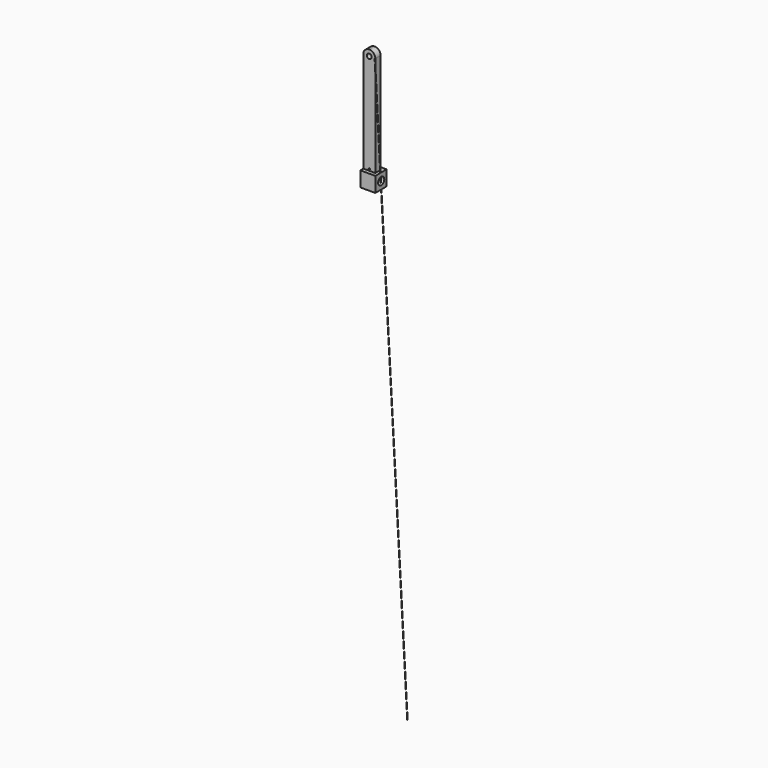
from build123d import *
from build123d import SkipClean  # not in build123d's __all__

# Parameters (mm, degrees)
F1_DEPTH      = 22
F2_R          = 8.15
F3_DEPTH      = 22.001
F3_TAPER      = 5.72
F4_W          = 40
F4_H          = 50
F5_DEPTH      = 12.5
F5_DEPTH_BACK = 34.5
F6_R          = 12.7
F7_DEPTH      = 40.001
F8_R          = 12.7
F9_DEPTH      = 10
F10_R         = 2.5
F11_DEPTH     = 25
F14_R         = 0.5
F15_DEPTH     = 2000


# Not quite as in the source:
# - after a boolean that leaves OpenCascade's solid faulty, fix() repairs it


with BuildPart() as f1:
    # F0 (on Front) → F1 (new body)
    with BuildSketch(Plane.XZ):
        with BuildLine():
            Line((0, 385), (0, 0))
            Line((0, 0), (40, 0))
            Line((40, 0), (40, 385))
            ThreePointArc((40, 385), (34.1421356237, 399.1421356237), (20, 405))
            ThreePointArc((20, 405), (5.8578643763, 399.1421356237), (0, 385))
        make_face()
    extrude(amount=F1_DEPTH)

    # F2 (on face) → F3 (cut, through all)
    with BuildSketch(Plane.XZ.offset(22)):
        with Locations((20, 385)):
            Circle(F2_R)
    extrude(amount=-F3_DEPTH, taper=F3_TAPER, mode=Mode.SUBTRACT)

    # F4 (on face) → F5 (join, two sides)
    with BuildSketch(Plane.XZ.offset(22)) as f5_sk:
        with Locations((20, 25)):
            Rectangle(F4_W, F4_H)
    extrude(amount=F5_DEPTH)
    extrude(f5_sk.sketch, amount=-F5_DEPTH_BACK)

    # F6 (on face) → F7 (cut, through all)
    with BuildSketch(Plane(origin=(0, 0, 0), x_dir=(0, -1, 0), z_dir=(-1, 0, 0))):
        with Locations((10, 25)):
            Circle(F6_R)
    extrude(amount=-F7_DEPTH, mode=Mode.SUBTRACT)

    # F8 (on face) → F9 (join)
    with BuildSketch(Plane.YZ.offset(40)):
        Polygon((0, 50), (-22, 50), (-34.5, 50), (-34.5, 0), (12.5, 0), (12.5, 50), align=None)
        with Locations((-10, 25)):
            Circle(F8_R, mode=Mode.SUBTRACT)
    with SkipClean():  # cleaning this boolean's faces spoils the solid; the shape is the same uncleaned
        extrude(amount=F9_DEPTH)

    # F10 (on face) → F11 (cut)
    with BuildSketch(Plane.XZ.offset(22)):
        with Locations((20, 55)):
            Circle(F10_R)
    extrude(amount=-F11_DEPTH, mode=Mode.SUBTRACT)

    add(f1.part.fix(), mode=Mode.REPLACE)

    # F14 (on line) → F15 (join)
    with BuildSketch(Plane(origin=(0, -26.8080383352, 393.2344937713), x_dir=(1, 0, 0), z_dir=(0, -0.0680152907, 0.9976842788))):
        with Locations((48.9524379373, -8.5178036243)):
            Circle(F14_R)
    extrude(amount=-F15_DEPTH)


solid = f1.part
